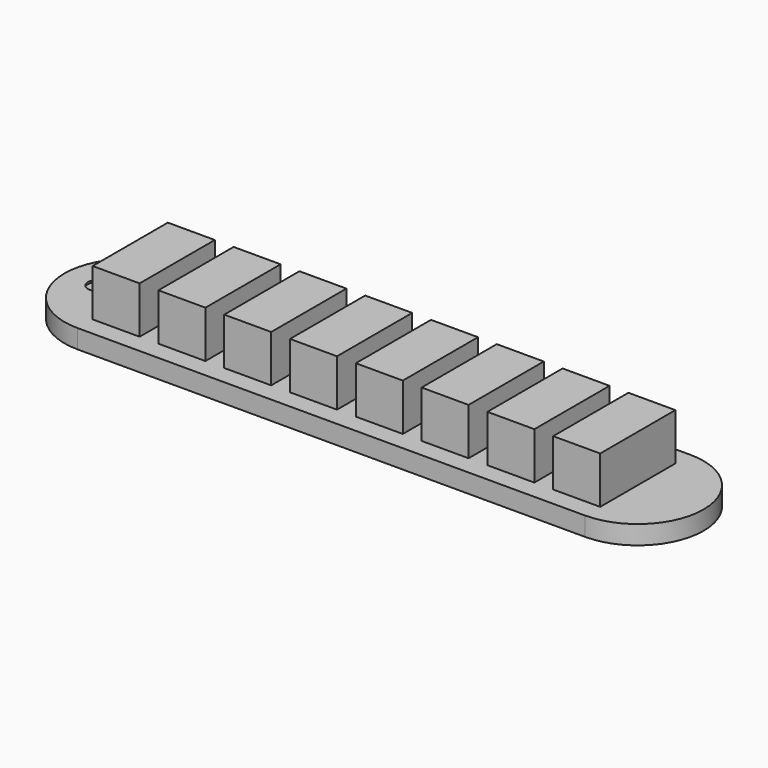
from build123d import *

# Parameters (mm, degrees)
F1_DEPTH = 1
F2_W     = 2.5
F2_H     = 5
F3_DEPTH = 2.5
F5_DEPTH = 0.1


# Not quite as in the source:
# - a feature names something its author has since deleted; it is built from what else it names


with BuildPart() as f1:
    # F0 (on Top) → F1 (new body)
    with BuildSketch(Plane.XY):
        with BuildLine():
            Line((0, 3.5), (-13.5, 3.5))
            ThreePointArc((-13.5, 3.5), (-17, 0), (-13.5, -3.5))
            Line((-13.5, -3.5), (0, -3.5))
            Line((0, -3.5), (13.5, -3.5))
            ThreePointArc((13.5, -3.5), (17, 0), (13.5, 3.5))
            Line((13.5, 3.5), (0, 3.5))
        make_face()
    extrude(amount=F1_DEPTH)

    # F2 (on face) → F3 (join)
    with BuildSketch(Plane.XY.offset(1)):
        with Locations((-12.25, 0)):
            Rectangle(F2_W, F2_H)
        with Locations((12.25, 0)):
            Rectangle(F2_W, F2_H)
        with Locations((-8.75, 0)):
            Rectangle(F2_W, F2_H)
        with Locations((-5.25, 0)):
            Rectangle(F2_W, F2_H)
        with Locations((-1.75, 0)):
            Rectangle(F2_W, F2_H)
        with Locations((1.75, 0)):
            Rectangle(F2_W, F2_H)
        with Locations((5.25, 0)):
            Rectangle(F2_W, F2_H)
        with Locations((8.75, 0)):
            Rectangle(F2_W, F2_H)
    extrude(amount=F3_DEPTH)

    # F4 (on face) → F5 (cut)
    with BuildSketch(Plane.XY.offset(1)):
        with BuildLine():
            ThreePointArc((-15.75, 0), (-15.25, -0.5), (-14.75, 0))
            ThreePointArc((-14.75, 0), (-15.25, 0.5), (-15.75, 0))
        make_face()
    extrude(amount=-F5_DEPTH, mode=Mode.SUBTRACT)


solid = f1.part
